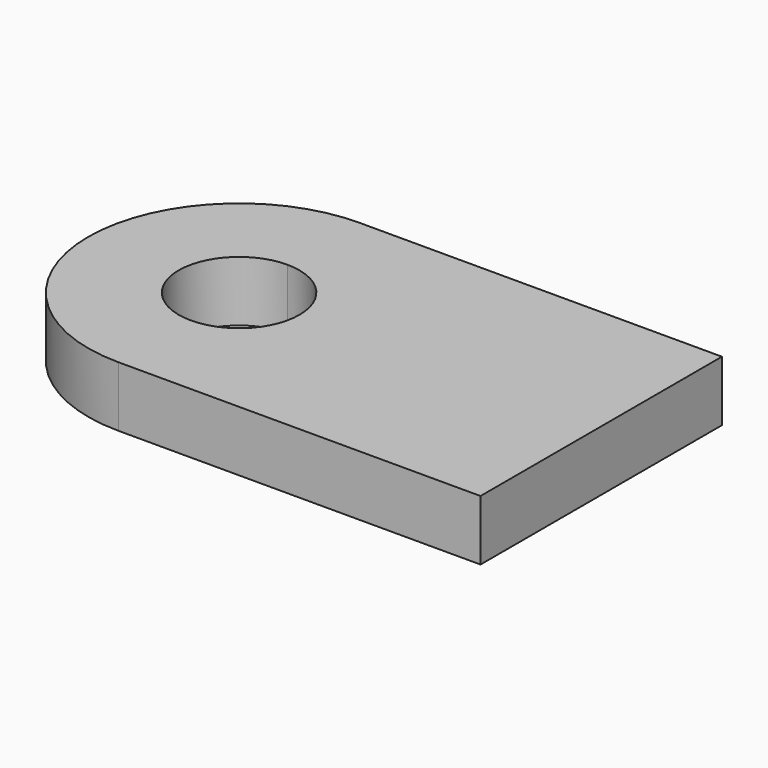
from build123d import *

# Parameters (mm, degrees)
F1_DEPTH = 12.7


# Not quite as in the source:
# - a feature of the source that left no trace in its solid (it failed there, or was rolled back) is left out


with BuildPart() as f1:
    # F0 (on Top) → F1 (new body)
    with BuildSketch(Plane.XY):
        with BuildLine():
            Line((-38.1, -31.75), (38.1, -31.75))
            Line((38.1, -31.75), (38.1, 31.75))
            Line((38.1, 31.75), (-38.1, 31.75))
            ThreePointArc((-38.1, 31.75), (-15.6493596973, 22.4506403027), (-6.35, 0))
            ThreePointArc((-6.35, 0), (-15.6493596973, -22.4506403027), (-38.1, -31.75))
        make_face()
        with BuildLine():
            ThreePointArc((-38.1, 31.75), (-69.85, 0), (-38.1, -31.75))
            Line((-38.1, -31.75), (-38.1, -12.7))
            ThreePointArc((-38.1, -12.7), (-50.8, 0), (-38.1, 12.7))
            Line((-38.1, 12.7), (-38.1, 31.75))
        make_face()
        with BuildLine():
            Line((-38.1, -12.7), (-38.1, -31.75))
            ThreePointArc((-38.1, -31.75), (-15.6493596973, -22.4506403027), (-6.35, 0))
            ThreePointArc((-6.35, 0), (-15.6493596973, 22.4506403027), (-38.1, 31.75))
            Line((-38.1, 31.75), (-38.1, 12.7))
            ThreePointArc((-38.1, 12.7), (-29.1197438789, 8.9802561211), (-25.4, 0))
            ThreePointArc((-25.4, 0), (-29.1197438789, -8.9802561211), (-38.1, -12.7))
        make_face()
    extrude(amount=F1_DEPTH)


solid = f1.part
